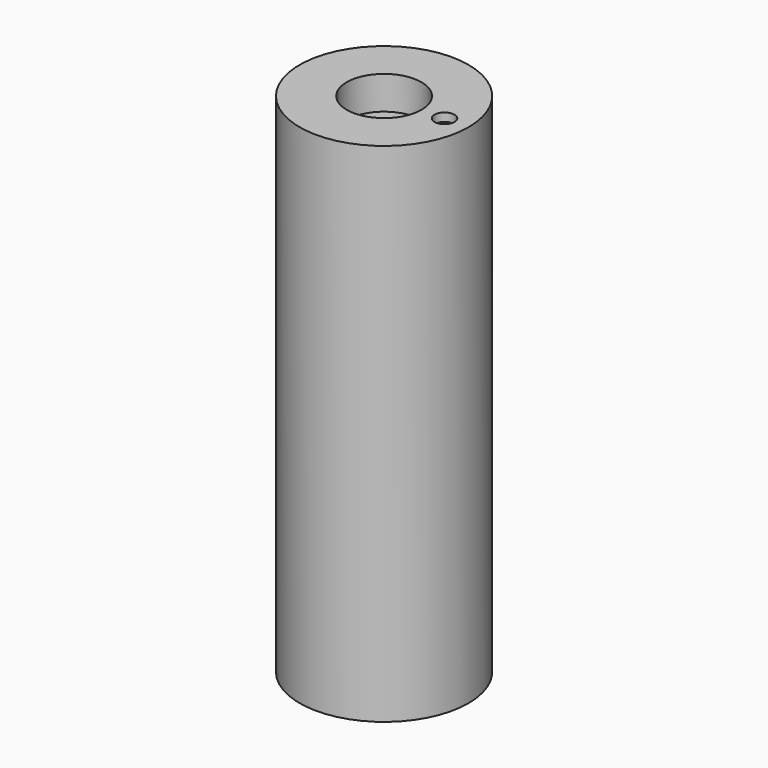
from build123d import *

# Parameters (mm, degrees)
F0_R      = 25.4
F1_DEPTH  = 152.5
F2_T      = -2.5
F3_R      = 6.5
F4_DEPTH  = 150
F5_T      = -2.5
F6_R      = 13.75
F7_DEPTH  = 12
F8_R      = 11.25
F11_DEPTH = 10
F12_R     = 25.4
F13_DEPTH = 2.5
F14_R     = 13.75
F15_DEPTH = 12.5
F16_R     = 11.25
F17_DEPTH = 10
F18_R     = 4
F19_DEPTH = 142.501
F20_R     = 3
F21_DEPTH = 25


# Not quite as in the source:
# - a fillet or chamfer that OpenCascade refuses, or shapes differently, is made with other operations: its cross-section is extruded or revolved along the edge and cut away or added


with BuildPart() as f1:
    # F0 (on Top) → F1 (new body)
    with BuildSketch(Plane.XY):
        Circle(F0_R)
    extrude(amount=F1_DEPTH)

    # F2
    f2_openings = [f1.faces().sort_by_distance(p)[0] for p in [
        (0, 0, 152.5),
    ]]
    offset(amount=F2_T, openings=f2_openings)

    # F3 (on face) → F4 (join)
    with BuildSketch(Plane.XY.offset(2.5)):
        Circle(F3_R)
    extrude(amount=F4_DEPTH)

    # F5: a shell. OpenCascade refuses it in one call, so the cavity is built on its own and cut out:
    # the body offset inwards by the wall thickness, plus a prism from it out through each open face.
    f5_core = offset(f1.part, amount=F5_T, kind=Kind.INTERSECTION, mode=Mode.PRIVATE)
    f5_exits = [f5_core.faces().sort_by_distance(p)[0] for p in [
        (0, 0, 150),
    ]]
    add(f5_core, mode=Mode.SUBTRACT)
    extrude(f5_exits, amount=-F5_T, mode=Mode.SUBTRACT)

    # F6 (on face) → F7 (join)
    with BuildSketch(Plane(origin=(0, 0, 0), x_dir=(1, 0, 0), z_dir=(0, 0, -1))):
        Circle(F6_R)
    extrude(amount=-F7_DEPTH)

    # F9: fillet of radius 10 on 1 edges, made by hand

    # F9_s1 → F9_t2 (revolve)
    with BuildSketch(Plane.XZ):
        with BuildLine():
            ThreePointArc((22.9, 12.4638095124), (20.2654599313, 5.6999348832), (13.75, 2.5))
            Line((13.75, 2.5), (22.9, 2.5))
            Line((22.9, 2.5), (22.9, 12.4638095124))
        make_face()
    revolve(axis=Axis((0, 0, 2.5), (0, 0, -1)))

    # F10: fillet of radius 8 on 1 edges, made by hand

    # F10_s1 → F10_t2 (revolve)
    with BuildSketch(Plane.XZ):
        with BuildLine():
            ThreePointArc((13.75, 12), (8.5839202169, 14.5796013539), (6.5, 19.964766161))
            Line((6.5, 19.964766161), (6.5, 12))
            Line((6.5, 12), (13.75, 12))
        make_face()
    revolve(axis=Axis((0, 0, 12), (0, 0, -1)))

    # F8 (on face) → F11 (cut)
    with BuildSketch(Plane(origin=(0, 0, 0), x_dir=(1, 0, 0), z_dir=(0, 0, -1))):
        Circle(F8_R)
    extrude(amount=-F11_DEPTH, mode=Mode.SUBTRACT)

    # F12 (on face) → F13 (join)
    with BuildSketch(Plane.XY.offset(152.5)):
        Circle(F12_R)
    extrude(amount=-F13_DEPTH)

    # F14 (on face) → F15 (join)
    with BuildSketch(Plane.XY.offset(152.5)):
        Circle(F14_R)
    extrude(amount=-F15_DEPTH)

    # F16 (on face) → F17 (cut)
    with BuildSketch(Plane.XY.offset(152.5)):
        Circle(F16_R)
    extrude(amount=-F17_DEPTH, mode=Mode.SUBTRACT)

    # F18 (on face) → F19 (cut, through all)
    with BuildSketch(Plane.XY.offset(142.5)):
        Circle(F18_R)
    extrude(amount=-F19_DEPTH, mode=Mode.SUBTRACT)

    # F20 (on face) → F21 (cut)
    with BuildSketch(Plane.XY.offset(152.5)):
        with Locations((18.1747831392, 0)):
            Circle(F20_R)
    extrude(amount=-F21_DEPTH, mode=Mode.SUBTRACT)


solid = f1.part
